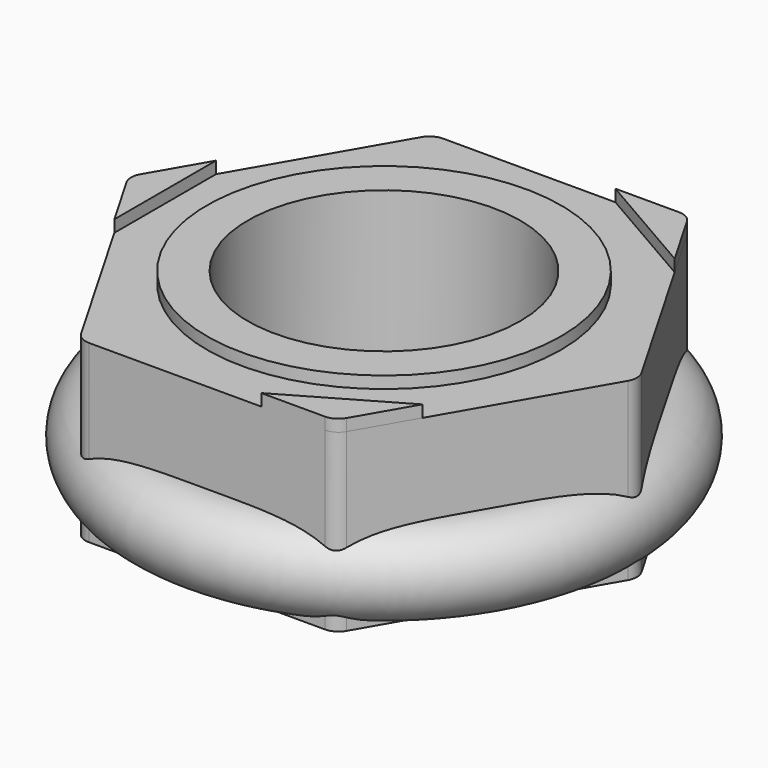
from build123d import *

# Parameters (mm, degrees)
F0_R            = 4
F1_DEPTH        = 5.15
F2_R            = 0.5
F4_DEPTH        = 0.35
F4_COPIES_COUNT = 3
F3_R            = 5.2
F3_R_2          = 4
F5_DEPTH        = 0.35


# Not quite as in the source:
# - a pattern or mirror of a feature is missing from the dataset's text; its kind, count and spacing are read off the source's solid


with BuildPart() as f1:
    # F0 (on Top) → F1 (new body)
    with BuildSketch(Plane.XY):
        Polygon((3.75, 6.4951905284), (-3.75, 6.4951905284), (-7.5, 0), (-3.75, -6.4951905284), (3.75, -6.4951905284), (7.5, 0), align=None)
        Circle(F0_R, mode=Mode.SUBTRACT)
    extrude(amount=F1_DEPTH)

    # F2
    f2_edges = [f1.edges().sort_by_distance(p)[0] for p in [
        (3.75, -6.495191, 2.575),
        (7.5, 0, 2.575),
        (3.75, 6.495191, 2.575),
        (-3.75, 6.495191, 2.575),
        (-7.5, 0, 2.575),
        (-3.75, -6.495191, 2.575),
    ]]
    fillet(f2_edges, radius=F2_R)

    # F3 (on face) → F4 (join)
    with BuildSketch(Plane.XY.offset(5.15)):
        with BuildLine():
            Line((-6.4226497308, 1.8660254038), (-7.3556624327, 0.25))
            ThreePointArc((-7.3556624327, 0.25), (-7.4226497308, 0), (-7.3556624327, -0.25))
            Line((-7.3556624327, -0.25), (-6.4226497308, -1.8660254038))
            Line((-6.4226497308, -1.8660254038), (-6.4226497308, 1.8660254038))
        make_face()
    f4 = extrude(amount=F4_DEPTH)

    # F4_copies: F4 ×3 about axis
    f4_copies_axis = Axis((0, 0, 0), (0, 0, 1))
    for i in range(1, F4_COPIES_COUNT):
        add(f4.rotate(f4_copies_axis, i * 360 / F4_COPIES_COUNT))

    # F3 (on face) → F5 (join, through all)
    with BuildSketch(Plane.XY.offset(5.15)):
        Circle(F3_R)
        Circle(F3_R_2, mode=Mode.SUBTRACT)
    extrude(amount=F5_DEPTH)

    # F6 (on Right) → F7 (revolve)
    with BuildSketch(Plane.YZ):
        with BuildLine():
            ThreePointArc((-6.4951905284, 2.5), (-7.7451905284, 1.25), (-6.4951905284, 0))
            Line((-6.4951905284, 0), (-6.4951905284, 2.5))
        make_face()
    revolve(axis=Axis((0, 0, -0.6419573572), (0, 0, -1)))


solid = f1.part
